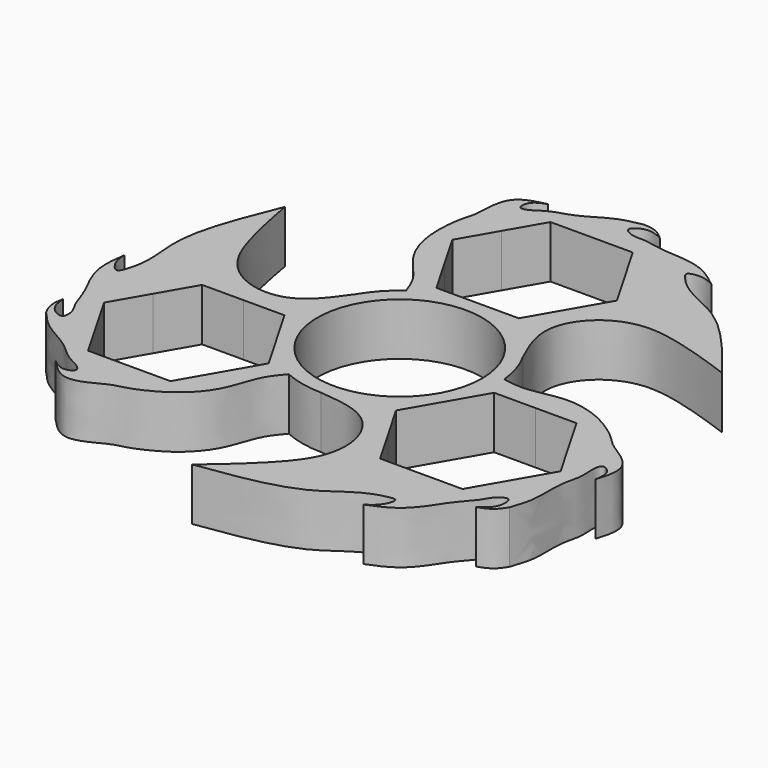
from build123d import *

# Parameters (mm, degrees)
F0_R     = 11
F1_DEPTH = 7
F2_COUNT = 3


# Not quite as in the source:
# - the dataset's text gives a spline's control points without its knots; the knots are read off the source's solid
# - a feature names something its author has since deleted; it is built from what else it names


with BuildPart() as f1:
    # F0 (on Top) → F1 (new body)
    with BuildSketch(Plane.XY):
        with BuildLine():
            ThreePointArc((-7.5919963353, 10.5528001803), (-5.9289142194, -11.5692686104), (13, 0))
            ThreePointArc((13, 0), (12.5704087578, 3.3143360817), (11.3100271289, 6.4096245088))
            ThreePointArc((11.3100271289, 6.4096245088), (6.5450317559, 11.2322107937), (-1.3e-09, 13))
            ThreePointArc((-1.3e-09, 13), (-3.9883328388, 12.3730837372), (-7.5919963353, 10.5528001803))
        make_face()
        Circle(F0_R, mode=Mode.SUBTRACT)
        with BuildLine():
            ThreePointArc((-1.3e-09, 13), (6.5450317559, 11.2322107937), (11.3100271289, 6.4096245088))
            add(Edge.make_bspline(
                [(11.3100271289, 6.4096245088), (10.8277603254, 7.4519494012), (9.8727913781, 9.5159316196), (9.101870084, 13.2022847878), (10.9930717603, 17.3935667079), (15.9445286102, 20.3038165496), (22.7412492325, 19.1222960129), (27.2302822076, 17.5269663637), (29.7399077416, 16.6350860483)],
                knots=[0, 0, 0, 0, 3.454281, 6.840065, 10.920147, 16.370579, 22.717522, 30.7646, 30.7646, 30.7646, 30.7646], degree=3))
            add(Edge.make_bspline(
                [(29.7399077416, 16.6350860483), (28.4836475385, 18.2461931845), (25.5987360843, 21.9450952017), (20.2017189577, 27.5050498478), (15.0428882075, 28.6673343945), (12.5690115148, 31.9385999614), (14.6811233168, 32.4518778122), (15.7083520351, 31.9192701431), (16.407615424, 31.5567081202)],
                knots=[0.0144537192, 0.0144537192, 0.0144537192, 0.0144537192, 6.194486, 14.203525, 22.074143, 22.873829, 24.051284, 26.561775, 26.561775, 26.561775, 26.561775], degree=3))
            add(Edge.make_bspline(
                [(16.407615424, 31.5567081202), (15.4049023222, 32.3399165847), (13.4658196059, 33.8535190511), (10.3452119002, 34.3357889044), (7.9344434577, 34.3971594843), (6.2147244404, 34.7080952785), (4.5063669183, 35.0713247495), (3.1082707439, 34.8574787663), (1.3380885049, 35.8789758676), (3.4983566078, 37.3892054026), (4.7888025313, 36.7817520454), (5.6452574026, 36.3785922272)],
                knots=[0.0046949721, 0.0046949721, 0.0046949721, 0.0046949721, 3.759757, 7.265106, 9.201956, 11.001497, 12.529867, 14.308463, 15.525968, 16.929978, 19.700717, 19.700717, 19.700717, 19.700717], degree=3))
            add(Edge.make_bspline(
                [(5.6452574026, 36.3785922272), (5.3176826436, 36.6663420667), (4.6978399336, 37.2108137216), (3.5549068491, 37.6517152685), (2.7918842622, 37.6775809796), (2.4171225183, 37.6902842884)],
                knots=[8.42234e-05, 8.42234e-05, 8.42234e-05, 8.42234e-05, 1.300895, 2.461477, 3.58171, 3.58171, 3.58171, 3.58171], degree=3))
            add(Edge.make_bspline(
                [(2.4171225183, 37.6902842884), (1.4466554473, 37.4993707055), (-0.4802140411, 37.1194555701), (-2.7454735423, 35.6953695532), (-4.66514216, 34.6570397494), (-6.2994083365, 34.2363899874), (-7.708171918, 33.604292052), (-8.6422176542, 32.8292069294), (-10.184834153, 32.3150830289), (-10.1833973742, 34.322673268), (-9.0410345214, 34.7536662817), (-8.2196646451, 35.0635532875)],
                knots=[0.0069720876, 0.0069720876, 0.0069720876, 0.0069720876, 2.946289, 5.843961, 7.960875, 9.446163, 10.927091, 12.421396, 13.511085, 14.446457, 16.839917, 16.839917, 16.839917, 16.839917], degree=3))
            add(Edge.make_bspline(
                [(-8.2196646451, 35.0635532875), (-9.6386773765, 34.7271226927), (-12.0399656, 34.1482725614), (-12.6960723373, 30.8024553033), (-12.6216866169, 28.5513207343), (-13.2601924534, 26.705797678), (-13.4613053983, 24.996943365), (-13.6667091736, 21.6575187534), (-12.5114237856, 16.9708953473), (-8.770627027, 13.7904170142), (-7.8878258097, 11.3654245815), (-7.5919963353, 10.5528001803)],
                knots=[0.027850683, 0.027850683, 0.027850683, 0.027850683, 3.977544, 6.733705, 9.242712, 10.828127, 12.508482, 14.390484, 20.894773, 25.990246, 28.558335, 28.558335, 28.558335, 28.558335], degree=3))
            ThreePointArc((-7.5919963353, 10.5528001803), (-3.9883328388, 12.3730837372), (-1.3e-09, 13))
        make_face()
        Polygon((5.499261314, 13), (-1.3e-09, 13), (-5.499261314, 13), (-8.2488920963, 17.7625002169), (-10.9985226281, 22.525), (-8.24889179, 27.2875003136), (-5.499261314, 32.05), (0, 32.05), (5.499261314, 32.05), (8.2488918485, 27.2875002122), (10.9985226281, 22.525), (8.248891917, 17.7624999064), align=None, mode=Mode.SUBTRACT)
    extrude(amount=F1_DEPTH)

    # F2: F1 ×3 about axis
    f2_axis = Axis((0, 0, 7), (0, 0, 1))


with BuildPart() as f1_1:
    add(f1.part)
    for i in range(1, F2_COUNT):
        add(f1.part.rotate(f2_axis, i * 360 / F2_COUNT))


solid = f1_1.part
